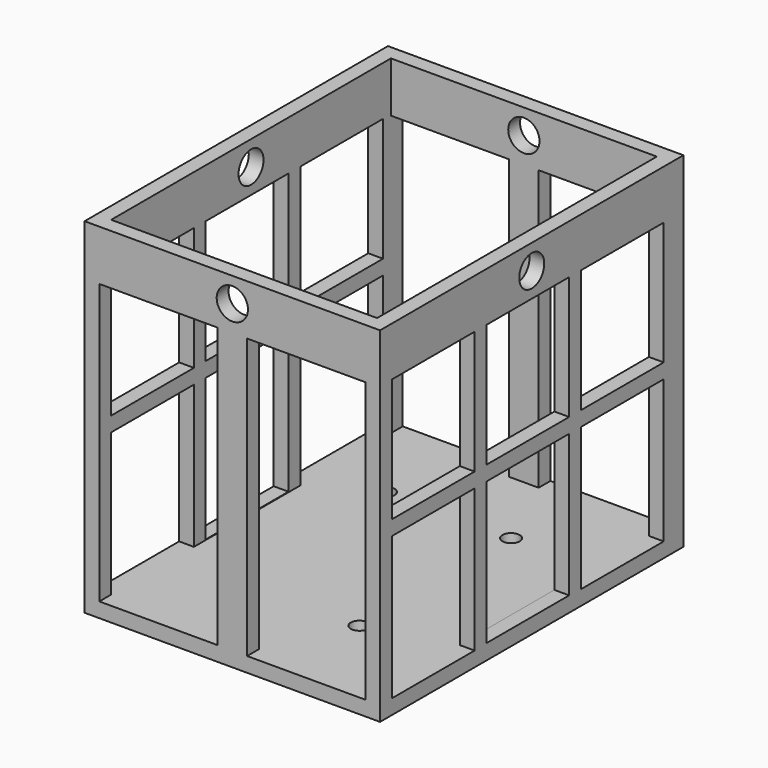
from build123d import *

# Parameters (mm, degrees)
F0_W      = 60
F0_H      = 77
F1_DEPTH  = 70
F2_T      = -3
F3_W      = 21
F3_H      = 25
F3_H_2    = 29
F3_H_3    = 28.8890717719
F4_DEPTH  = 60.001
F5_R      = 1.75
F6_DEPTH  = 3.001
F3_R      = 3.175
F7_DEPTH  = 60.001
F8_R      = 3.175
F8_W      = 24
F8_H      = 56.7587303836
F9_DEPTH  = 77.001
F10_DEPTH = 77.001


# Not quite as in the source:
# - a feature names something its author has since deleted; it is built from what else it names


with BuildPart() as f1:
    # F0 (on Top) → F1 (new body)
    with BuildSketch(Plane.XY):
        Rectangle(F0_W, F0_H)
    extrude(amount=F1_DEPTH)

    # F2
    f2_openings = [f1.faces().sort_by_distance(p)[0] for p in [
        (0, 0, 70),
    ]]
    offset(amount=F2_T, openings=f2_openings)

    # F3 (on face) → F4 (cut, through all)
    with BuildSketch(Plane.YZ.offset(30)):
        with Locations((-25, 47.5)):
            Rectangle(F3_W, F3_H)
        with Locations((-1, 47.5)):
            Rectangle(F3_W, F3_H)
        with Locations((23, 47.5)):
            Rectangle(F3_W, F3_H)
        with Locations((-25, 17.5)):
            Rectangle(F3_W, F3_H_2)
        with Locations((-1, 17.5554641141)):
            Rectangle(F3_W, F3_H_3)
        with Locations((23, 17.5)):
            Rectangle(F3_W, F3_H_2)
    extrude(amount=-F4_DEPTH, mode=Mode.SUBTRACT)

    # F5 (on face) → F6 (cut, through all)
    with BuildSketch(Plane.XY.offset(3)):
        with Locations((-15, -19.25)):
            Circle(F5_R)
        with Locations((10.4, -19.25)):
            Circle(F5_R)
        with Locations((-15, 19.25)):
            Circle(F5_R)
        with Locations((10.4, 19.25)):
            Circle(F5_R)
    extrude(amount=-F6_DEPTH, mode=Mode.SUBTRACT)

    # F3 (on face) → F7 (cut, through all)
    with BuildSketch(Plane.YZ.offset(30)):
        with Locations((0, 65)):
            Circle(F3_R)
    extrude(amount=-F7_DEPTH, mode=Mode.SUBTRACT)

    # F8 (on face) → F9 (cut, through all)
    with BuildSketch(Plane(origin=(0, 38.5, 0), x_dir=(-1, 0, 0), z_dir=(0, 1, 0))):
        with Locations((0, 65)):
            Circle(F8_R)
        with Locations((-15, 31.3793651918)):
            Rectangle(F8_W, F8_H)
        with Locations((15, 31.3793651918)):
            Rectangle(F8_W, F8_H)
    extrude(amount=-F9_DEPTH, mode=Mode.SUBTRACT)

    # F8 (on face) → F10 (cut, through all)
    with BuildSketch(Plane(origin=(0, 38.5, 0), x_dir=(-1, 0, 0), z_dir=(0, 1, 0))):
        with Locations((0, 65)):
            Circle(F8_R)
        with Locations((-15, 31.3793651918)):
            Rectangle(F8_W, F8_H)
        with Locations((15, 31.3793651918)):
            Rectangle(F8_W, F8_H)
    extrude(amount=-F10_DEPTH, mode=Mode.SUBTRACT)


solid = f1.part
